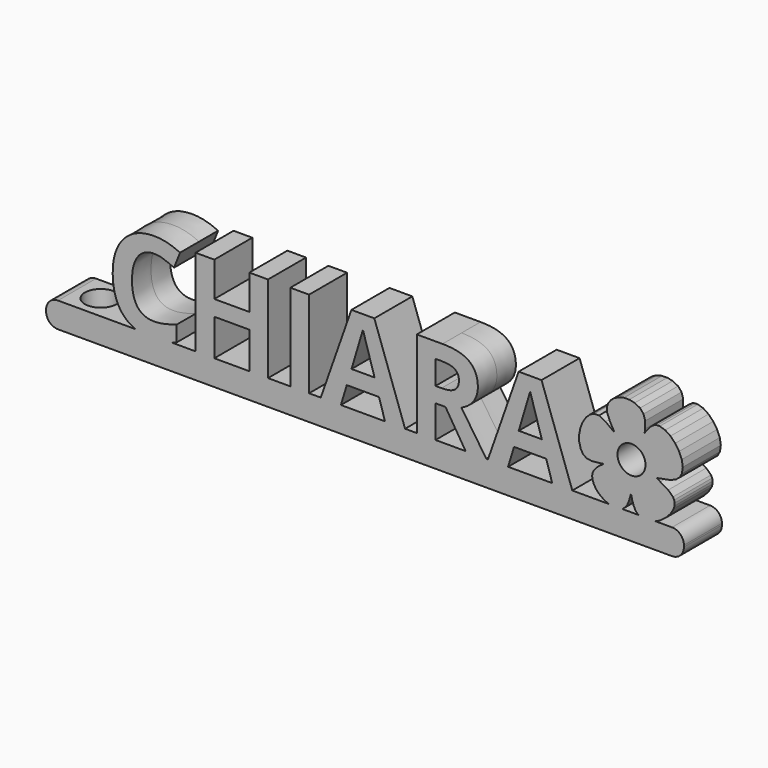
from build123d import *

# Parameters (mm, degrees)
F0_R         = 1.7660260944
F0_TEXT_SIZE = 15.6313604168
F1_DEPTH     = 3
F2_W         = 73
F2_H         = 6
F3_DEPTH     = 0.2
F4_DEPTH     = 3
F5_W         = 6
F5_H         = 3.2
F6_DEPTH     = 7.5
F7_R         = 1.5
F8_R         = 2
F9_DEPTH     = 4
F10_R        = 1.5


# Not quite as in the source:
# - Text() gives the source's letters only with a copy of the font that has no kerning and outlines rounded to 1/6400 em; it was checked with that copy


with BuildPart() as f1:
    # F0 (on Front) → F1 (new body, symmetric)
    with BuildSketch(Plane.XZ):
        Polygon((48.6077747296, -0.0299610052), (49.1946776084, 0.099542717), (49.9729476218, 0.4643786716), (50.715370662, 1.015622925), (51.3286791697, 1.6703047302), (51.7195851589, 2.3454487056), (51.8195518667, 2.6977360466), (51.8387514567, 3.0240118137), (51.7727665329, 3.3305925609), (51.6171796484, 3.6238062012), (51.0195032111, 4.1953846239), (50.010366981, 4.7892998886), (49.5765909733, 5.0567831223), (50.0858876127, 5.1580765572), (51.1908791002, 5.3695361343), (51.9559022863, 5.6521941309), (52.4516482732, 6.0438513785), (52.7487877368, 6.5823040735), (52.8619022613, 7.3346827269), (52.7288763332, 8.1369111543), (52.395029396, 8.9328580798), (51.9056899604, 9.6663968117), (51.3061660599, 10.2814073825), (50.6417771383, 10.7217585164), (49.9578448805, 10.9313257632), (49.6227117473, 10.9320269584), (49.299686438, 10.8539823803), (48.8570928163, 10.5612859992), (48.36391613, 9.9810365666), (48.0531798532, 9.5801643811), (48.097170502, 10.0271686186), (48.1123734909, 10.9311556967), (47.9055596605, 11.6324206604), (47.4676675691, 12.148064371), (46.7896380163, 12.4951945154), (46.1057383266, 12.6383143231), (45.4327625175, 12.6247534784), (44.8007719618, 12.4733706745), (44.2398075556, 12.203031329), (43.7799306718, 11.8325941351), (43.4511799144, 11.3809290439), (43.2836166564, 10.8668947486), (43.3072886194, 10.3093544253), (43.6753458761, 9.4077545298), (44.1510212197, 8.5454740537), (44.2133826416, 8.4004773751), (44.0228346252, 8.5293859694), (43.1093202517, 9.2300893731), (42.2859709356, 9.6332436777), (41.7009565662, 9.6341217666), (41.1471527001, 9.3699869944), (40.6514768597, 8.8932531607), (40.2408351574, 8.2563453735), (39.9421496489, 7.5116797243), (39.7823309803, 6.7116836131), (39.7882943817, 5.908775373), (39.9869482577, 5.1553755785), (40.3031060465, 4.6439943924), (40.7527626382, 4.3560669615), (41.3953792004, 4.2712955843), (42.2904167997, 4.3694052776), (42.7995414082, 4.4302814209), (42.8342995909, 4.4000046444), (42.7249732847, 4.3290259531), (42.3388523247, 4.0708069127), (41.9516788892, 3.7127982124), (41.6368875732, 3.3322638906), (41.4679129717, 3.0064679853), (41.4208892237, 2.6043627827), (41.4800682951, 2.1921007752), (41.6363740395, 1.7819255057), (41.8807120754, 1.386094067), (42.2039926052, 1.0168544849), (42.5971235394, 0.6864593188), (43.0510173725, 0.4071520608), (43.5565864978, 0.1911989214), (44.0642448882, 0.0570082487), (44.5199082953, 0.018892615), (44.9242654598, 0.0772799287), (45.2780322734, 0.2326232097), (45.5819020609, 0.4853412996), (45.8365861803, 0.8358849261), (46.0427847317, 1.2846820482), (46.2012022978, 1.8321742764), (46.3160204733, 2.2557758394), (46.3730871728, 2.0998483299), (46.4927724422, 1.5291341921), (46.6802150418, 0.9902805094), (46.908581132, 0.546686851), (47.1510369237, 0.261741427), (47.5518870373, 0.0538434116), (48.048822828, -0.0442882514), align=None)
        with Locations((46.3854075562, 6.0541478503)):
            Circle(F0_R, mode=Mode.SUBTRACT)
        with Locations((-20, 0)):
            Text('CHIARA', F0_TEXT_SIZE, font='Open Sans', font_style=FontStyle.BOLD, text_align=(TextAlign.LEFT, TextAlign.BOTTOM))
    extrude(amount=F1_DEPTH, both=True)



with BuildPart() as f3:
    # F2 (on Top) → F3 (new body)
    with BuildSketch(Plane.XY):
        with Locations((16.5, 0)):
            Rectangle(F2_W, F2_H)
    extrude(amount=F3_DEPTH)


with BuildPart() as f4:
    # F4 (new): a face of the model
    f4_faces = [f3.part.faces().sort_by_distance(p)[0] for p in [
        (16.5, 0, 0),
    ]]
    extrude(f4_faces, amount=F4_DEPTH)


with BuildPart() as f1_1:
    add(f1.part)

    add(f3.part)  # F6 merges F3

    add(f4.part)  # F6 merges F4
    # F5 (on face) → F6 (join)
    with BuildSketch(Plane(origin=(-20, 0, 0), x_dir=(0, -1, 0), z_dir=(-1, 0, 0))):
        with Locations((0, -1.4)):
            Rectangle(F5_W, F5_H)
    extrude(amount=F6_DEPTH)

    # F7
    f7_edges = [f1_1.edges().sort_by_distance(p)[0] for p in [
        (-27.5, 0, -3),
        (-27.5, 0, 0.2),
        (53, 0, -3),
    ]]
    fillet(f7_edges, radius=F7_R)

    # F8 (on face) → F9 (cut)
    with BuildSketch(Plane.XY.offset(0.2)):
        with Locations((-23, 0)):
            Circle(F8_R)
    extrude(amount=-F9_DEPTH, mode=Mode.SUBTRACT)

    # F10
    f10_edges = [f1_1.edges().sort_by_distance(p)[0] for p in [
        (53, 0, 0.2),
    ]]
    fillet(f10_edges, radius=F10_R)


solid = f1_1.part
